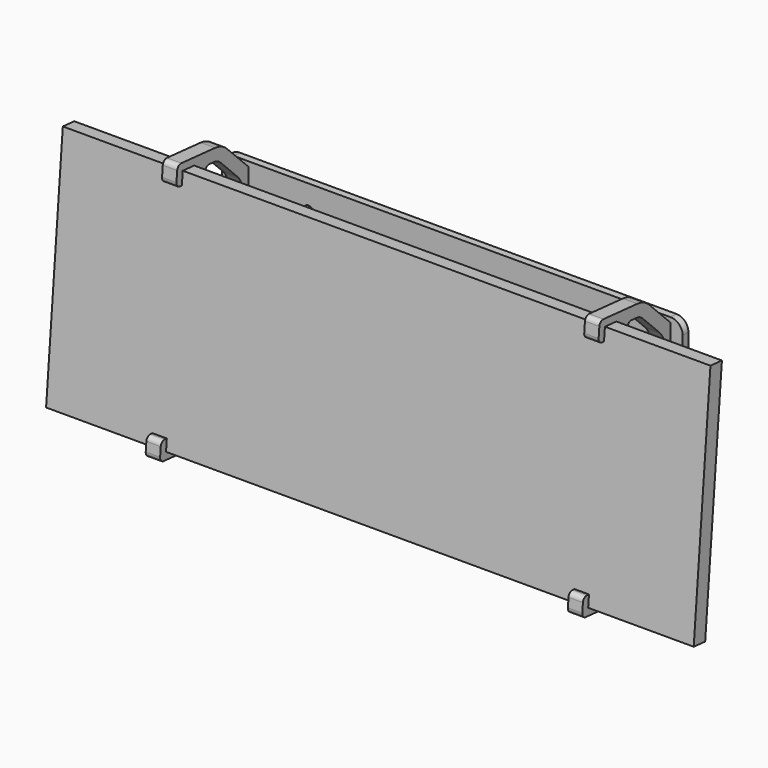
from build123d import *

# Parameters (mm, degrees)
F2_W      = 270
F2_H      = 100
F3_DEPTH  = 6
F6_DEPTH  = 6
F8_R      = 10
F8_2_R    = 10
F8_3_R    = 10
F8_4_R    = 10
F9_R      = 2
F9_2_R    = 2
F9_3_R    = 2
F9_4_R    = 2
F10_W     = 192
F10_H     = 84.9170803202
F10_W_2   = 6
F10_H_2   = 8.3333333333
F10_R     = 2
F11_DEPTH = 3
F12_R     = 5
F14_DEPTH = 703


with BuildPart() as f3:
    # F2 (on line) → F3 (new body)
    with BuildSketch(Plane(origin=(0, 0, 0), x_dir=(-1, 0, 0), z_dir=(0, 0.9961946981, -0.0871557427))):
        Rectangle(F2_W, F2_H)
    extrude(amount=F3_DEPTH)


with BuildPart() as f6:
    # F5 (on offset) → F6 (new body)
    with BuildSketch(Plane(origin=(-85, 0, 0), x_dir=(0, -1, 0), z_dir=(-1, 0, 0))):
        with BuildLine():
            Line((-3.8974684014, 44.5482676763), (-0.9088843071, 44.8097349046))
            Line((-0.9088843071, 44.8097349046), (-1.6306702714, 53.0597862271))
            Line((-1.6306702714, 53.0597862271), (-21.2518680197, 51.3431538593))
            ThreePointArc((-21.2518680197, 51.3431538593), (-24.5958757045, 50.4492282053), (-27.4347958571, 48.46881844))
            Line((-27.4347958571, 48.46881844), (-41.6193810512, 34.350529596))
            Line((-41.6193810512, 34.350529596), (-41.6193810512, 26.0171962627))
            Line((-41.6193810512, 26.0171962627), (-38.6193810512, 26.0171962627))
            Line((-38.6193810512, 26.0171962627), (-38.6193810512, 17.6838629293))
            Line((-38.6193810512, 17.6838629293), (-41.6193810512, 17.6838629293))
            Line((-41.6193810512, 17.6838629293), (-41.6193810512, 9.350529596))
            Line((-41.6193810512, 9.350529596), (-35.6193810512, 9.350529596))
            Line((-35.6193810512, 9.350529596), (-35.6193810512, 33.2679239334))
            Line((-35.6193810512, 33.2679239334), (-23.9075532246, 44.9250126592))
            ThreePointArc((-23.9075532246, 44.9250126592), (-22.4880931483, 45.9152175418), (-20.8160893059, 46.3621803689))
            Line((-20.8160893059, 46.3621803689), (-17.0290202972, 46.6935059751))
            Line((-17.0290202972, 46.6935059751), (-14.8556100804, 43.5895545061))
            Line((-14.8556100804, 43.5895545061), (-9.8746365899, 44.0253332199))
            Line((-9.8746365899, 44.0253332199), (-10.3349553259, 49.2868004481))
            Line((-10.3349553259, 49.2868004481), (-4.3577871374, 49.8097349046))
            Line((-4.3577871374, 49.8097349046), (-3.8974684014, 44.5482676763))
        make_face()
    extrude(amount=F6_DEPTH)


with BuildPart() as f6b:
    # F5 (on offset) → F6, piece 2 (new body)
    with BuildSketch(Plane(origin=(-85, 0, 0), x_dir=(0, -1, 0), z_dir=(-1, 0, 0))):
        with BuildLine():
            Line((6.9318033324, -44.8097349046), (3.9432192381, -45.0712021328))
            Line((3.9432192381, -45.0712021328), (4.3577871374, -49.8097349046))
            Line((4.3577871374, -49.8097349046), (-1.6193810512, -50.3326693611))
            Line((-1.6193810512, -50.3326693611), (-2.0339489504, -45.5941365893))
            Line((-2.0339489504, -45.5941365893), (-7.0149224409, -46.0299153031))
            Line((-7.0149224409, -46.0299153031), (-8.3601526442, -48.9147707838))
            Line((-8.3601526442, -48.9147707838), (-13.8382536726, -49.3940425214))
            ThreePointArc((-13.8382536726, -49.3940425214), (-15.3237410956, -49.3016385176), (-16.7162154514, -48.7760659227))
            Line((-16.7162154514, -48.7760659227), (-35.6193810512, -38.1950382371))
            Line((-35.6193810512, -38.1950382371), (-35.6193810512, -15.5665507242))
            Line((-35.6193810512, -15.5665507242), (-41.6193810512, -15.5665507242))
            Line((-41.6193810512, -15.5665507242), (-41.6193810512, -23.8998840575))
            Line((-41.6193810512, -23.8998840575), (-38.6193810512, -23.8998840575))
            Line((-38.6193810512, -23.8998840575), (-38.6193810512, -32.2332173909))
            Line((-38.6193810512, -32.2332173909), (-41.6193810512, -32.2332173909))
            Line((-41.6193810512, -32.2332173909), (-41.6193810512, -40.5665507242))
            Line((-41.6193810512, -40.5665507242), (-19.1583985164, -53.1390628144))
            ThreePointArc((-19.1583985164, -53.1390628144), (-16.3734498049, -54.1902080042), (-13.4024749589, -54.3750160119))
            Line((-13.4024749589, -54.3750160119), (7.6078384599, -52.5368517706))
            Line((7.6078384599, -52.5368517706), (6.9318033324, -44.8097349046))
        make_face()
    extrude(amount=F6_DEPTH)


with BuildPart() as f7_1:
    # F7: instance of F6
    add(f6.part.mirror(Plane.YZ))

    # F8#3
    f8_3_edges = [f7_1.edges().sort_by_distance(p)[0] for p in [
        (88, 35.619381, 33.267924),
    ]]
    fillet(f8_3_edges, radius=F8_3_R)

    # F9#3
    f9_3_edges = [f7_1.edges().sort_by_distance(p)[0] for p in [
        (88, 35.619381, 9.35053),
        (88, 1.63067, 53.059786),
        (88, 0.908884, 44.809735),
        (88, 17.02902, 46.693506),
        (88, 14.85561, 43.589555),
    ]]
    fillet(f9_3_edges, radius=F9_3_R)


with BuildPart() as f7_2:
    # F7: instance of F6b
    add(f6b.part.mirror(Plane.YZ))

    # F8#4
    f8_4_edges = [f7_2.edges().sort_by_distance(p)[0] for p in [
        (88, 35.619381, -38.195038),
    ]]
    fillet(f8_4_edges, radius=F8_4_R)

    # F9#4
    f9_4_edges = [f7_2.edges().sort_by_distance(p)[0] for p in [
        (88, 7.014922, -46.029915),
        (88, 8.360153, -48.914771),
        (88, 35.619381, -15.566551),
        (88, -6.931803, -44.809735),
        (88, -7.607838, -52.536852),
    ]]
    fillet(f9_4_edges, radius=F9_4_R)


with BuildPart() as f6_1:
    add(f6.part)

    # F8
    f8_edges = [f6_1.edges().sort_by_distance(p)[0] for p in [
        (-88, 35.619381, 33.267924),
    ]]
    fillet(f8_edges, radius=F8_R)

    # F9
    f9_edges = [f6_1.edges().sort_by_distance(p)[0] for p in [
        (-88, 35.619381, 9.35053),
        (-88, 1.63067, 53.059786),
        (-88, 0.908884, 44.809735),
        (-88, 17.02902, 46.693506),
        (-88, 14.85561, 43.589555),
    ]]
    fillet(f9_edges, radius=F9_R)


with BuildPart() as f6b_1:
    add(f6b.part)

    # F8#2
    f8_2_edges = [f6b_1.edges().sort_by_distance(p)[0] for p in [
        (-88, 35.619381, -38.195038),
    ]]
    fillet(f8_2_edges, radius=F8_2_R)

    # F9#2
    f9_2_edges = [f6b_1.edges().sort_by_distance(p)[0] for p in [
        (-88, 35.619381, -15.566551),
        (-88, -6.931803, -44.809735),
        (-88, -7.607838, -52.536852),
        (-88, 8.360153, -48.914771),
        (-88, 7.014922, -46.029915),
    ]]
    fillet(f9_2_edges, radius=F9_2_R)


with BuildPart() as f11:
    # F10 (on face) → F11 (new body)
    with BuildSketch(Plane(origin=(0, 38.6193810512, 0), x_dir=(-1, 0, 0), z_dir=(0, 1, 0))):
        with Locations((0, -3.1080105641)):
            Rectangle(F10_W, F10_H)
        with Locations((-88, -36.3998840575)):
            Rectangle(F10_W_2, F10_H_2, mode=Mode.SUBTRACT)
        with Locations((-60, -30.3326693611)):
            Circle(F10_R, mode=Mode.SUBTRACT)
        with Locations((-88, -19.7332173909)):
            Rectangle(F10_W_2, F10_H_2, mode=Mode.SUBTRACT)
        with Locations((88, -36.3998840575)):
            Rectangle(F10_W_2, F10_H_2, mode=Mode.SUBTRACT)
        with Locations((60, -30.3326693611)):
            Circle(F10_R, mode=Mode.SUBTRACT)
        with Locations((88, -19.7332173909)):
            Rectangle(F10_W_2, F10_H_2, mode=Mode.SUBTRACT)
        with Locations((-88, 13.5171962627)):
            Rectangle(F10_W_2, F10_H_2, mode=Mode.SUBTRACT)
        with Locations((-88, 30.1838629293)):
            Rectangle(F10_W_2, F10_H_2, mode=Mode.SUBTRACT)
        with Locations((-60, 29.2868004481)):
            Circle(F10_R, mode=Mode.SUBTRACT)
        with Locations((88, 13.5171962627)):
            Rectangle(F10_W_2, F10_H_2, mode=Mode.SUBTRACT)
        with Locations((60, 29.2868004481)):
            Circle(F10_R, mode=Mode.SUBTRACT)
        with Locations((88, 30.1838629293)):
            Rectangle(F10_W_2, F10_H_2, mode=Mode.SUBTRACT)
    extrude(amount=F11_DEPTH)

    # F12
    f12_edges = [f11.edges().sort_by_distance(p)[0] for p in [
        (96, 40.119381, 39.35053),
        (96, 40.119381, -45.566551),
        (-96, 40.119381, -45.566551),
        (-96, 40.119381, 39.35053),
    ]]
    fillet(f12_edges, radius=F12_R)


with BuildPart() as f14_tool:
    # F13 (on face) → F14 (new body)
    with BuildSketch(Plane(origin=(-91, 0, 0), x_dir=(0, -1, 0), z_dir=(-1, 0, 0))):
        Polygon((-38.6193810512, 40.4036790133), (-43.4263913442, 34.350529596), (-38.6193810512, 34.350529596), align=None)
        Polygon((-38.6193810512, -40.5665507242), (-45.0114011765, -40.5665507242), (-38.6193810512, -48.2738559767), align=None)
    extrude(amount=-F14_DEPTH)


with BuildPart() as f6_2:
    add(f6_1.part)

    # F14: cut by f14_tool
    add(f14_tool.part, mode=Mode.SUBTRACT)


with BuildPart() as f6b_2:
    add(f6b_1.part)

    # F14: cut by f14_tool
    add(f14_tool.part, mode=Mode.SUBTRACT)


with BuildPart() as f7_1_1:
    add(f7_1.part)

    # F14: cut by f14_tool
    add(f14_tool.part, mode=Mode.SUBTRACT)


with BuildPart() as f7_2_1:
    add(f7_2.part)

    # F14: cut by f14_tool
    add(f14_tool.part, mode=Mode.SUBTRACT)


solid = Compound([f3.part, f11.part, f6_2.part, f6b_2.part, f7_1_1.part, f7_2_1.part])
